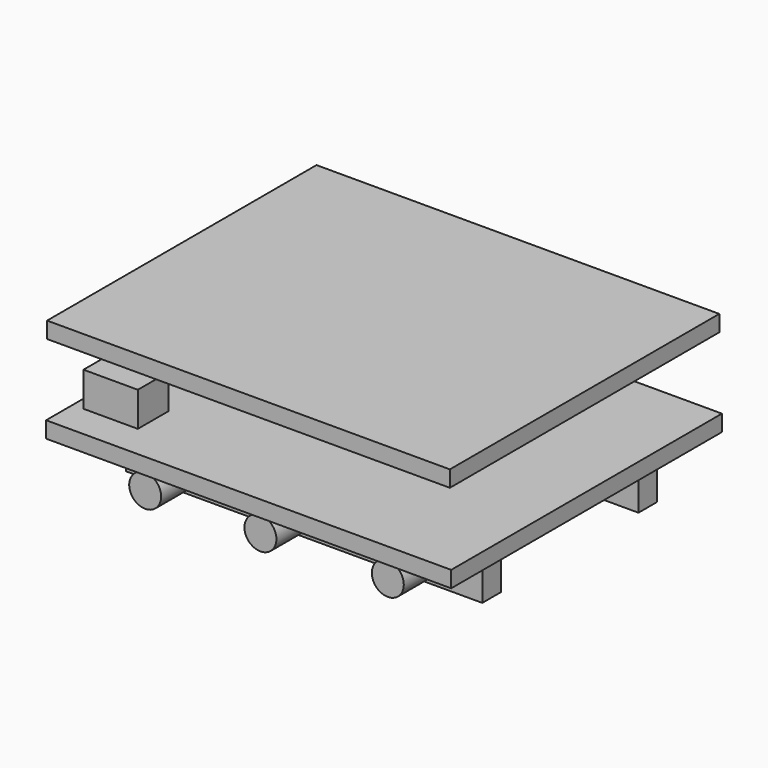
from build123d import *

# Parameters (mm, degrees)
F0_W          = 63.3566528559
F0_H          = 52.9265124351
F1_DEPTH      = 2.54
F2_W          = 52.6668075472
F2_H          = 2.5405590422
F3_DEPTH      = 29.972
F3_DEPTH_BACK = 33.02
F4_W          = 55.6830130517
F4_H          = 3.6676051095
F5_DEPTH      = 7.62
F6_R          = 2.498100457
F7_DEPTH      = 25.4
F7_DEPTH_BACK = 25.4
F8_W          = 26.8697123975
F8_H          = 5.2229278954
F9_DEPTH      = 25.4
F9_DEPTH_BACK = 25.4
F10_W         = 8.5002798587
F10_H         = 6.0210302472
F11_DEPTH     = 7.9248


# Not quite as in the source:
# - the program builds the solid bodies; features that only make, move or delete a surface that nothing else refers to are left out


with BuildPart() as f1:
    # F0 (on Top) → F1 (new body)
    with BuildSketch(Plane.XY):
        with Locations((1.5970468521, -1.6539534554)):
            Rectangle(F0_W, F0_H)
    extrude(amount=F1_DEPTH)

    # F4 (on Top) → F5 (join)
    with BuildSketch(Plane.XY):
        with Locations((1.6654524952, -15.4954805039)):
            Rectangle(F4_W, F4_H)
        with Locations((1.6654524952, 15.0418034755)):
            Rectangle(F4_W, F4_H)
    extrude(amount=-F5_DEPTH)

    # F6 (on Front) → F7 (join, two sides)
    with BuildSketch(Plane.XZ) as f7_sk:
        with Locations((21.1912784725, -3.7213952746)):
            Circle(F6_R)
        with Locations((-16.7551450431, -3.9340448566)):
            Circle(F6_R)
        with Locations((1.2700000079, -3.9340448566)):
            Circle(F6_R)
    extrude(amount=F7_DEPTH)
    extrude(f7_sk.sketch, amount=-F7_DEPTH_BACK)

    # F8 (on Right) → F9 (cut, two sides)
    with BuildSketch(Plane.YZ) as f9_sk:
        with Locations((-0.226829201, -3.8340105093)):
            Rectangle(F8_W, F8_H)
    extrude(amount=-F9_DEPTH, mode=Mode.SUBTRACT)
    extrude(f9_sk.sketch, amount=F9_DEPTH_BACK, mode=Mode.SUBTRACT)


with BuildPart() as f3:
    # F2 (on Right) → F3 (new body, two sides)
    with BuildSketch(Plane.YZ) as f3_sk:
        with Locations((-1.722917892, 14.9993023369)):
            Rectangle(F2_W, F2_H)
    extrude(amount=-F3_DEPTH)
    extrude(f3_sk.sketch, amount=F3_DEPTH_BACK)


with BuildPart() as f11:
    # F10 (on Top) → F11 (new body)
    with BuildSketch(Plane.XY):
        with Locations((-24.1524232551, -19.89361085)):
            Rectangle(F10_W, F10_H)
    extrude(amount=F11_DEPTH)


solid = Compound([f1.part, f3.part, f11.part])
